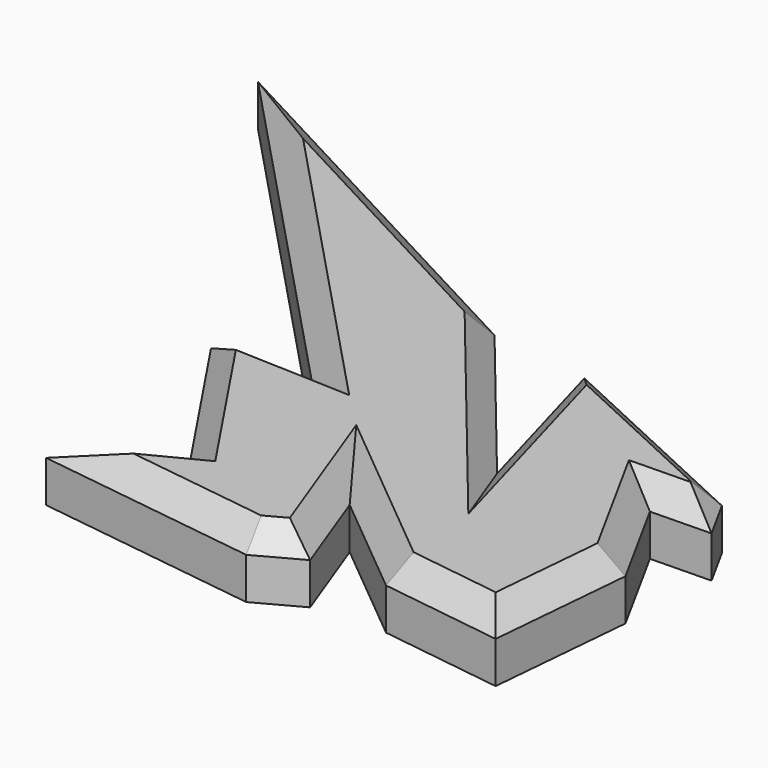
from build123d import *

# Parameters (mm, degrees)
F1_DEPTH = 12.7
F2_SIZE  = 4.572


# Not quite as in the source:
# - a feature names something its author has since deleted; it is built from what else it names


with BuildPart() as f1:
    # F0 (on Top) → F1 (new body)
    with BuildSketch(Plane.XY):
        Polygon((-47.4197901785, 9.0821487829), (-54.1167072952, 27.1118637174), (-33.1560820341, 9.7886463627), (-9.0490672737, 6.4328033477), (-6.5208841115, 34.9811986089), (-16.9482622296, 54.0015585721), (-5.0941226073, 54.2380437255), (-9.5673697069, 62.3648315668), (-52.2826313972, 82.1464285254), (-43.0134832859, 49.2380969226), (-71.8594374871, 84.6780897401), (-152.3833320228, 127.5459273348), (-82.3831111193, 53.5424649715), (-102.9803976417, 54.3163046241), (-80.3189948201, 20.4314347357), (-100.0030711293, 10.3000625968), (-56.1285279691, 4.3535600416), align=None)
    extrude(amount=F1_DEPTH)

    # F2
    f2_edges = [f1.edges().sort_by_distance(p)[0] for p in [
        (-30.925001, 72.25563, 12.7),
        (-47.648057, 65.692263, 12.7),
        (-57.43646, 66.958093, 12.7),
        (-112.121385, 106.112009, 12.7),
        (-117.383222, 90.544196, 12.7),
        (-92.681754, 53.929385, 12.7),
        (-91.649696, 37.37387, 12.7),
        (-90.161033, 15.365749, 12.7),
        (-78.0658, 7.326811, 12.7),
        (-51.774159, 6.717854, 12.7),
        (-50.768249, 18.097006, 12.7),
        (-43.636395, 18.450255, 12.7),
        (-21.102575, 8.110725, 12.7),
        (-7.784976, 20.707001, 12.7),
        (-11.734573, 44.491379, 12.7),
        (-11.021192, 54.119801, 12.7),
        (-7.330746, 58.301438, 12.7),
    ]]
    chamfer(f2_edges, length=F2_SIZE)


solid = f1.part
